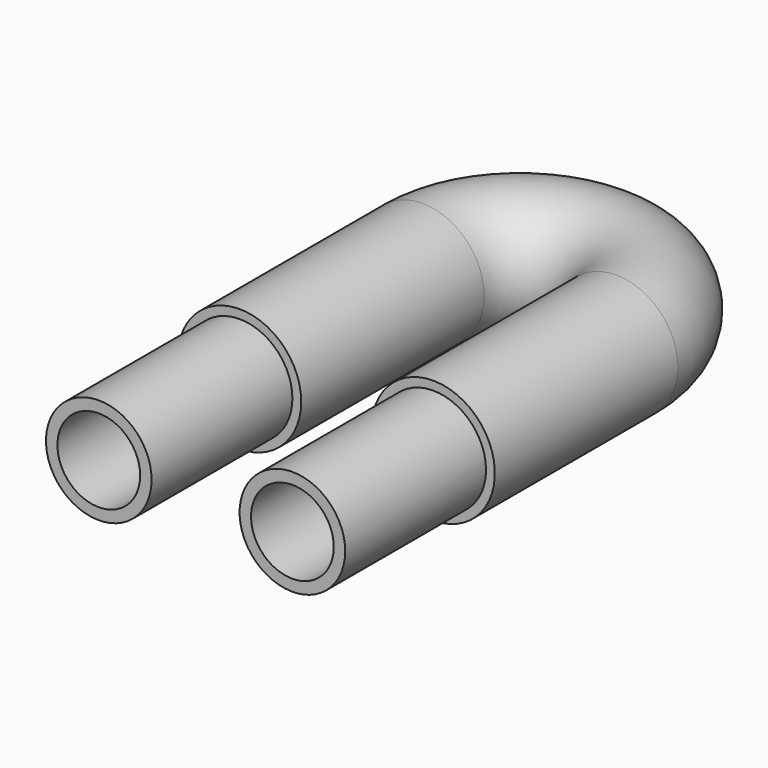
from build123d import *
from build123d import SkipClean  # not in build123d's __all__

# Parameters (mm, degrees)
F0_R     = 8.89
F0_R_2   = 5.969
F3_R     = 7.62
F3_R_2   = 5.969
F4_R     = 7.62
F4_R_2   = 5.969
F5_DEPTH = 25.4


with BuildPart() as f2:
    # F2: sweep along a path in F1
    with BuildLine(Plane.XY) as f2_path:
        Line((0, 0), (0, 33.02))
        ThreePointArc((0, 33.02), (13.97, 46.99), (27.94, 33.02))
        Line((27.94, 33.02), (27.94, 0))
    # F0 (on Front) → F2 (sweep)
    with BuildSketch(Plane.XZ):
        Circle(F0_R)
        Circle(F0_R_2, mode=Mode.SUBTRACT)
    sweep(path=f2_path.line)

    # F3 (on face) + F4 (on face) → F5 (join)
    with BuildSketch(Plane.XZ):
        Circle(F3_R)
        Circle(F3_R_2, mode=Mode.SUBTRACT)
    with BuildSketch(Plane.XZ):
        with Locations((27.94, 0)):
            Circle(F4_R)
        with Locations((27.94, 0)):
            Circle(F4_R_2, mode=Mode.SUBTRACT)
    with SkipClean():  # cleaning this boolean's faces spoils the solid; the shape is the same uncleaned
        extrude(amount=F5_DEPTH)


solid = f2.part
